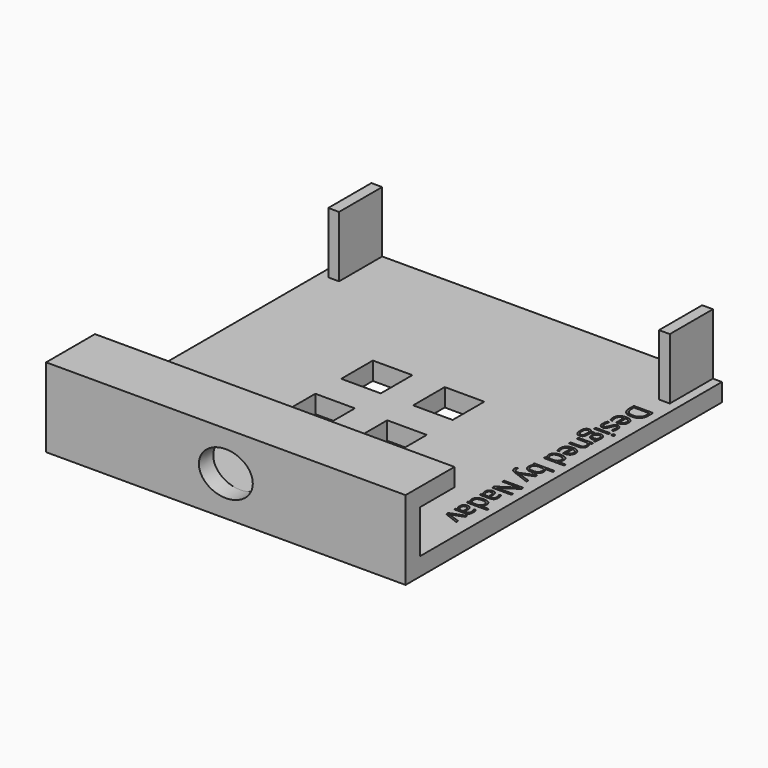
from build123d import *

# Parameters (mm, degrees)
F0_W         = 100
F0_H         = 110
F0_W_2       = 11
F0_H_2       = 11
F1_DEPTH     = 5
F2_W         = 3
F2_H         = 15
F2_W_2       = 100
F2_H_2       = 5
F3_DEPTH     = 17
F5_DEPTH     = 12
F6_DEPTH     = 25
F7_TEXT_SIZE = 7.5248551915
F8_DEPTH     = 1


# Not quite as in the source:
# - Text() gives the source's letters only with a copy of the font that has no kerning and outlines rounded to 1/6400 em; it was checked with that copy


with BuildPart() as f1:
    # F0 (on Top) → F1 (new body)
    with BuildSketch(Plane.XY):
        Rectangle(F0_W, F0_H)
        with Locations((-10, -10)):
            Rectangle(F0_W_2, F0_H_2, mode=Mode.SUBTRACT)
        with Locations((10, -10)):
            Rectangle(F0_W_2, F0_H_2, mode=Mode.SUBTRACT)
        with Locations((-10, 10)):
            Rectangle(F0_W_2, F0_H_2, mode=Mode.SUBTRACT)
        with Locations((10, 10)):
            Rectangle(F0_W_2, F0_H_2, mode=Mode.SUBTRACT)
    extrude(amount=F1_DEPTH)

    # F2 (on face) → F3 (join)
    with BuildSketch(Plane.XY.offset(5)):
        with Locations((-46, 47.5)):
            Rectangle(F2_W, F2_H)
        with Locations((46, 47.5)):
            Rectangle(F2_W, F2_H)
        with Locations((0, -52.5)):
            Rectangle(F2_W_2, F2_H_2)
    extrude(amount=F3_DEPTH)

    # F4 (on face) → F5 (join)
    with BuildSketch(Plane(origin=(0, -50, 0), x_dir=(-1, 0, 0), z_dir=(0, 1, 0))):
        Polygon((-1.95e-08, 17), (50, 17), (50, 22), (-50, 22), (-50, 17), align=None)
    extrude(amount=F5_DEPTH)

    # F4 (on face) → F6 (cut)
    with BuildSketch(Plane(origin=(0, -50, 0), x_dir=(-1, 0, 0), z_dir=(0, 1, 0))):
        with BuildLine():
            add(Edge.make_bspline(
                [(6.39e-08, 5), (7.5000000417, 5.0000000511), (7.5, 11.0000000333), (7.4999999583, 17.0000000156), (-1.95e-08, 17)],
                knots=[1.5707963353, 1.5707963353, 1.5707963353, 3.1415926591, 3.1415926591, 4.712388983, 4.712388983, 4.712388983], degree=2, weights=[1, 0.7071067822, 1, 0.7071067822, 1]))
            add(Edge.make_bspline(
                [(-1.95e-08, 17), (-7.5, 16.9999999844), (-7.5, 11)],
                knots=[4.712388983, 4.712388983, 4.712388983, 6.2831853072, 6.2831853072, 6.2831853072], degree=2, weights=[1, 0.7071067821, 1]))
            add(Edge.make_bspline(
                [(-7.5, 11), (-7.5, 4.9999999489), (6.39e-08, 5)],
                knots=[0, 0, 0, 1.5707963353, 1.5707963353, 1.5707963353], degree=2, weights=[1, 0.7071067782, 1]))
        make_face()
    extrude(amount=-F6_DEPTH, mode=Mode.SUBTRACT)

    # F7 (on face) → F8 (cut)
    with BuildSketch(Plane.XY.offset(5)):
        with Locations(Location((42.0821042621, 35), (0, 0, -90))):
            Text('Designed by Nadav', F7_TEXT_SIZE, font='Open Sans', text_align=(TextAlign.LEFT, TextAlign.BOTTOM))
    extrude(amount=-F8_DEPTH, mode=Mode.SUBTRACT)


solid = f1.part
